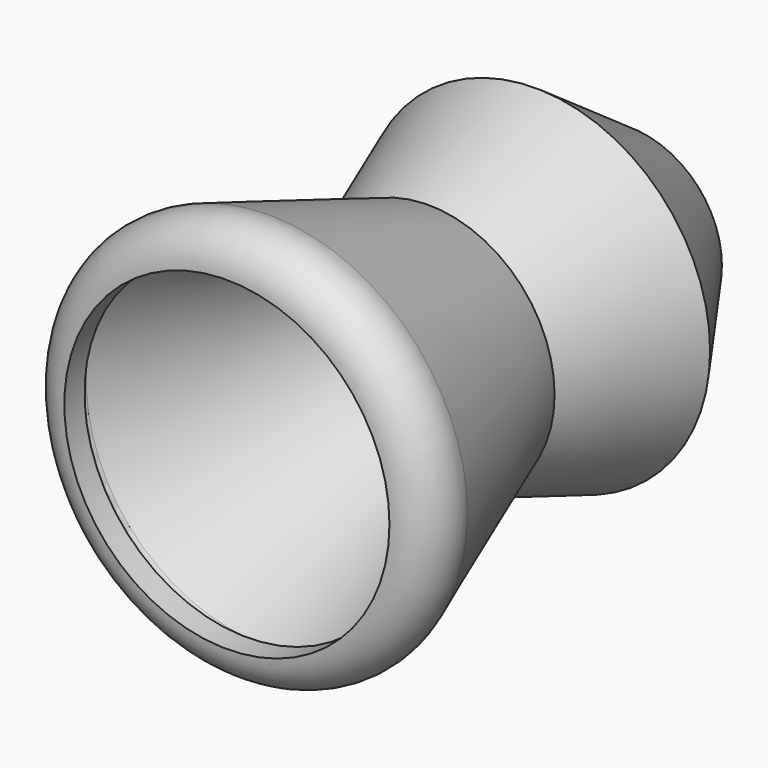
from build123d import *

# Parameters (mm, degrees)
F0_R     = 63.5
F1_DEPTH = 127
F1_TAPER = -20
F2_R     = 19.4741575124
F3_SIZE  = 63.5
F4_T     = -12.7


# Not quite as in the source:
# - a shell that OpenCascade refuses in one call is made with other operations: the cavity is built on its own and cut out


with BuildPart() as f1:
    # F0 (on Front) → F1 (new body, symmetric)
    with BuildSketch(Plane.XZ):
        Circle(F0_R)
    extrude(amount=F1_DEPTH, both=True, taper=F1_TAPER)

    # F2
    f2_edges = [f1.edges().sort_by_distance(p)[0] for p in [
        (-109.72422, -127, 0),
    ]]
    fillet(f2_edges, radius=F2_R)

    # F3
    f3_edges = [f1.edges().sort_by_distance(p)[0] for p in [
        (-109.72422, 127, 0),
    ]]
    chamfer(f3_edges, length=F3_SIZE)

    # F4: a shell. OpenCascade refuses it in one call, so the cavity is built on its own and cut out:
    # the body offset inwards by the wall thickness, plus a prism from it out through each open face.
    f4_core = offset(f1.part, amount=F4_T, kind=Kind.INTERSECTION, mode=Mode.PRIVATE)
    f4_exits = [f4_core.faces().sort_by_distance(p)[0] for p in [
        (0, -114.3, 0),
    ]]
    add(f4_core, mode=Mode.SUBTRACT)
    extrude(f4_exits, amount=-F4_T, mode=Mode.SUBTRACT)


solid = f1.part
